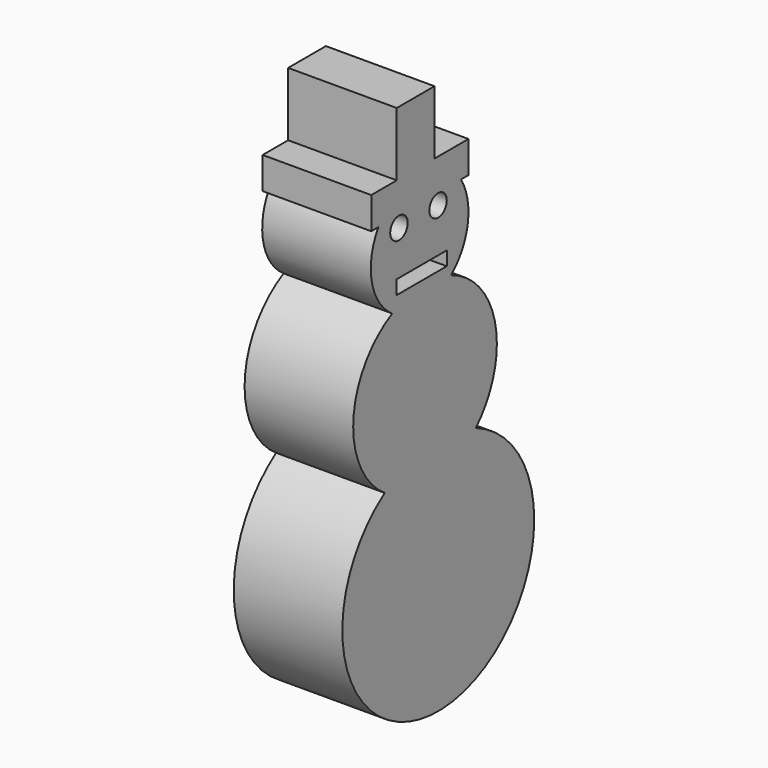
from build123d import *

# Parameters (mm, degrees)
F0_W     = 11.0358623788
F0_H     = 14.8984193802
F1_DEPTH = 25.4
F2_DEPTH = 25.4
F3_R     = 2.5571153932
F3_R_2   = 2.5440351013
F3_W     = 14.7031287464
F3_H     = 3.2673614761
F4_DEPTH = 25.4


# Not quite as in the source:
# - the program builds the solid bodies; features that only make, move or delete a surface that nothing else refers to are left out


with BuildPart() as f1:
    # F0 (on Right) → F1 (new body)
    with BuildSketch(Plane.YZ):
        with BuildLine():
            ThreePointArc((-24.4896995825, -21.3687317689), (-22.0066937129, -69.3902825337), (19.2165729762, -44.633931036))
            ThreePointArc((19.2165729762, -44.633931036), (14.5664371428, -29.167684068), (2.1580914014, -18.8302997515))
            ThreePointArc((2.1580914014, -18.8302997515), (-10.7088530026, -24.8964679727), (-24.4896995825, -21.3687317689))
        make_face()
        with BuildLine():
            ThreePointArc((-24.4896995825, -21.3687317689), (-10.7088530026, -24.8964679727), (2.1580914014, -18.8302997515))
            ThreePointArc((2.1580914014, -18.8302997515), (-11.4882033251, -16.7150534797), (-24.4896995825, -21.3687317689))
        make_face()
        with BuildLine():
            ThreePointArc((-24.4896995825, -21.3687317689), (-11.4882033251, -16.7150534797), (2.1580914014, -18.8302997515))
            ThreePointArc((2.1580914014, -18.8302997515), (6.7017838768, -12.0221001394), (8.2971597307, -3.993931036))
            ThreePointArc((8.2971597307, -3.993931036), (4.6343580327, 7.8551511373), (-5.0761488644, 15.5702610153))
            ThreePointArc((-5.0761488644, 15.5702610153), (-13.5382573111, 12.2302712352), (-22.2995232661, 14.6803793882))
            ThreePointArc((-22.2995232661, 14.6803793882), (-33.6585141964, -2.7205891991), (-24.4896995825, -21.3687317689))
        make_face()
        with BuildLine():
            ThreePointArc((-26.3456820786, 34.106068964), (-28.2496986989, 23.5752529976), (-22.2995232661, 14.6803793882))
            ThreePointArc((-22.2995232661, 14.6803793882), (-13.7834170108, 16.9752588467), (-5.0761488644, 15.5702610153))
            ThreePointArc((-5.0761488644, 15.5702610153), (-1.3310983759, 20.4668881546), (0, 26.486068964))
            ThreePointArc((0, 26.486068964), (-0.5620509112, 30.4522310833), (-2.2039436985, 34.106068964))
            Line((-2.2039436985, 34.106068964), (-26.3456820786, 34.106068964))
        make_face()
        with BuildLine():
            ThreePointArc((-5.0761488644, 15.5702610153), (-13.7834170108, 16.9752588467), (-22.2995232661, 14.6803793882))
            ThreePointArc((-22.2995232661, 14.6803793882), (-13.5382573111, 12.2302712352), (-5.0761488644, 15.5702610153))
        make_face()
        with BuildLine():
            Line((-28.4173451364, 34.106068964), (-26.3456820786, 34.106068964))
            ThreePointArc((-26.3456820786, 34.106068964), (-14.2748128886, 40.7608818526), (-2.2039436985, 34.106068964))
            Line((-2.2039436985, 34.106068964), (0, 34.106068964))
            Line((0, 34.106068964), (0, 41.5552749288))
            Line((0, 41.5552749288), (-9.9322767928, 41.5552749288))
            Line((-9.9322767928, 41.5552749288), (-20.9681391716, 41.5552749288))
            Line((-20.9681391716, 41.5552749288), (-28.4173451364, 41.5552749288))
            Line((-28.4173451364, 41.5552749288), (-28.4173451364, 34.106068964))
        make_face()
        with BuildLine():
            ThreePointArc((-2.2039436985, 34.106068964), (-14.2748128886, 40.7608818526), (-26.3456820786, 34.106068964))
            Line((-26.3456820786, 34.106068964), (-2.2039436985, 34.106068964))
        make_face()
        with Locations((-15.4502079822, 49.0044846189)):
            Rectangle(F0_W, F0_H)
    extrude(amount=F1_DEPTH)

    # F0 (on Right) → F2 (join)
    with BuildSketch(Plane.YZ):
        with BuildLine():
            ThreePointArc((-24.4896995825, -21.3687317689), (-22.0066937129, -69.3902825337), (19.2165729762, -44.633931036))
            ThreePointArc((19.2165729762, -44.633931036), (14.5664371428, -29.167684068), (2.1580914014, -18.8302997515))
            ThreePointArc((2.1580914014, -18.8302997515), (-10.7088530026, -24.8964679727), (-24.4896995825, -21.3687317689))
        make_face()
        with BuildLine():
            ThreePointArc((-24.4896995825, -21.3687317689), (-10.7088530026, -24.8964679727), (2.1580914014, -18.8302997515))
            ThreePointArc((2.1580914014, -18.8302997515), (-11.4882033251, -16.7150534797), (-24.4896995825, -21.3687317689))
        make_face()
        with BuildLine():
            ThreePointArc((-24.4896995825, -21.3687317689), (-11.4882033251, -16.7150534797), (2.1580914014, -18.8302997515))
            ThreePointArc((2.1580914014, -18.8302997515), (6.7017838768, -12.0221001394), (8.2971597307, -3.993931036))
            ThreePointArc((8.2971597307, -3.993931036), (4.6343580327, 7.8551511373), (-5.0761488644, 15.5702610153))
            ThreePointArc((-5.0761488644, 15.5702610153), (-13.5382573111, 12.2302712352), (-22.2995232661, 14.6803793882))
            ThreePointArc((-22.2995232661, 14.6803793882), (-33.6585141964, -2.7205891991), (-24.4896995825, -21.3687317689))
        make_face()
        with BuildLine():
            ThreePointArc((-26.3456820786, 34.106068964), (-28.2496986989, 23.5752529976), (-22.2995232661, 14.6803793882))
            ThreePointArc((-22.2995232661, 14.6803793882), (-13.7834170108, 16.9752588467), (-5.0761488644, 15.5702610153))
            ThreePointArc((-5.0761488644, 15.5702610153), (-1.3310983759, 20.4668881546), (0, 26.486068964))
            ThreePointArc((0, 26.486068964), (-0.5620509112, 30.4522310833), (-2.2039436985, 34.106068964))
            Line((-2.2039436985, 34.106068964), (-26.3456820786, 34.106068964))
        make_face()
        with BuildLine():
            ThreePointArc((-5.0761488644, 15.5702610153), (-13.7834170108, 16.9752588467), (-22.2995232661, 14.6803793882))
            ThreePointArc((-22.2995232661, 14.6803793882), (-13.5382573111, 12.2302712352), (-5.0761488644, 15.5702610153))
        make_face()
        with BuildLine():
            Line((-28.4173451364, 34.106068964), (-26.3456820786, 34.106068964))
            ThreePointArc((-26.3456820786, 34.106068964), (-14.2748128886, 40.7608818526), (-2.2039436985, 34.106068964))
            Line((-2.2039436985, 34.106068964), (0, 34.106068964))
            Line((0, 34.106068964), (0, 41.5552749288))
            Line((0, 41.5552749288), (-9.9322767928, 41.5552749288))
            Line((-9.9322767928, 41.5552749288), (-20.9681391716, 41.5552749288))
            Line((-20.9681391716, 41.5552749288), (-28.4173451364, 41.5552749288))
            Line((-28.4173451364, 41.5552749288), (-28.4173451364, 34.106068964))
        make_face()
        with BuildLine():
            ThreePointArc((-2.2039436985, 34.106068964), (-14.2748128886, 40.7608818526), (-26.3456820786, 34.106068964))
            Line((-26.3456820786, 34.106068964), (-2.2039436985, 34.106068964))
        make_face()
        with Locations((-15.4502079822, 49.0044846189)):
            Rectangle(F0_W, F0_H)
    extrude(amount=F2_DEPTH)

    # F3 (on Right) → F4 (cut)
    with BuildSketch(Plane.YZ):
        with Locations((-20.32, 31.496)):
            Circle(F3_R)
        with Locations((-8.89, 31.4950787105)):
            Circle(F3_R_2)
        with Locations((-13.7015643732, 19.5692073871)):
            Rectangle(F3_W, F3_H)
    extrude(amount=F4_DEPTH, mode=Mode.SUBTRACT)


solid = f1.part
